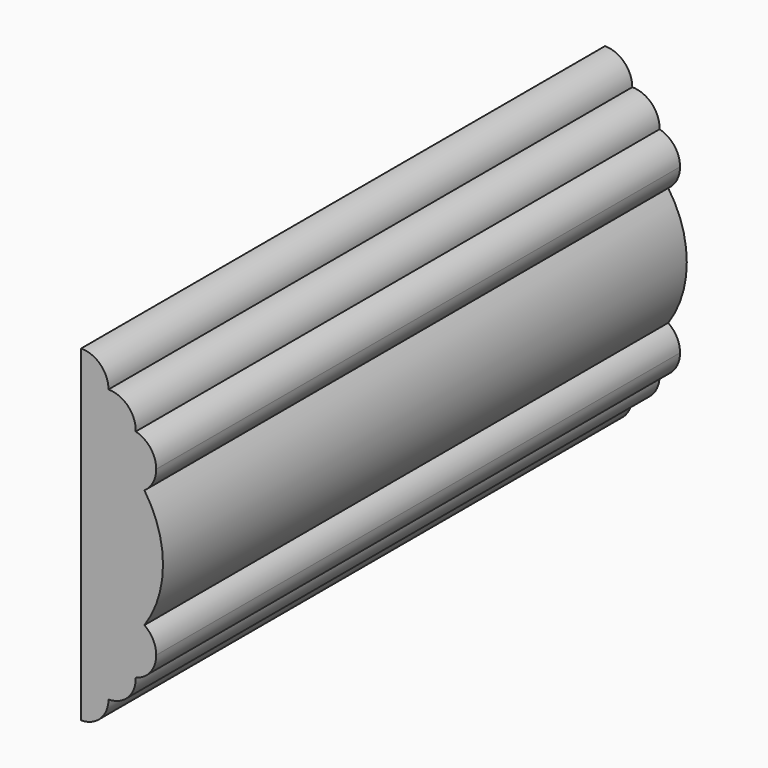
from build123d import *

# Parameters (mm, degrees)
F1_DEPTH = 152.4


# Not quite as in the source:
# - ends of sketch curves that miss each other by under 0.0002 mm in the source are joined


with BuildPart() as f1:
    # F0 (on Front) → F1 (new body)
    with BuildSketch(Plane.XZ):
        with BuildLine():
            ThreePointArc((-3.173984, 31.7550292), (-5.034153519, 36.245875681), (-9.525, 38.1060452))
            Line((-9.525, 38.1060452), (-9.525, -38.1060452))
            ThreePointArc((-9.525, -38.1060452), (-5.034153519, -36.245875681), (-3.173984, -31.7550292))
            ThreePointArc((-3.173984, -31.7550292), (1.3873070975, -29.8232975079), (3.1738358164, -25.2031917651))
            ThreePointArc((3.1738358164, -25.2031917651), (6.6091861803, -22.9435143548), (7.940294, -19.0530226))
            ThreePointArc((7.940294, -19.0530226), (7.2093686546, -16.094985199), (5.1848340025, -13.817816657))
            ThreePointArc((5.1848340025, -13.817816657), (9.5132844595, -8.141e-06), (5.1848116567, 13.8177933751))
            ThreePointArc((5.1848116567, 13.8177933751), (7.2093653059, 16.0949788365), (7.940294, 19.0530226))
            ThreePointArc((7.940294, 19.0530226), (6.6091861803, 22.9435143548), (3.1738358164, 25.2031917651))
            ThreePointArc((3.1738358164, 25.2031917651), (1.3873169736, 29.8232821056), (-3.173984, 31.7550292))
        make_face()
    extrude(amount=F1_DEPTH)


solid = f1.part
